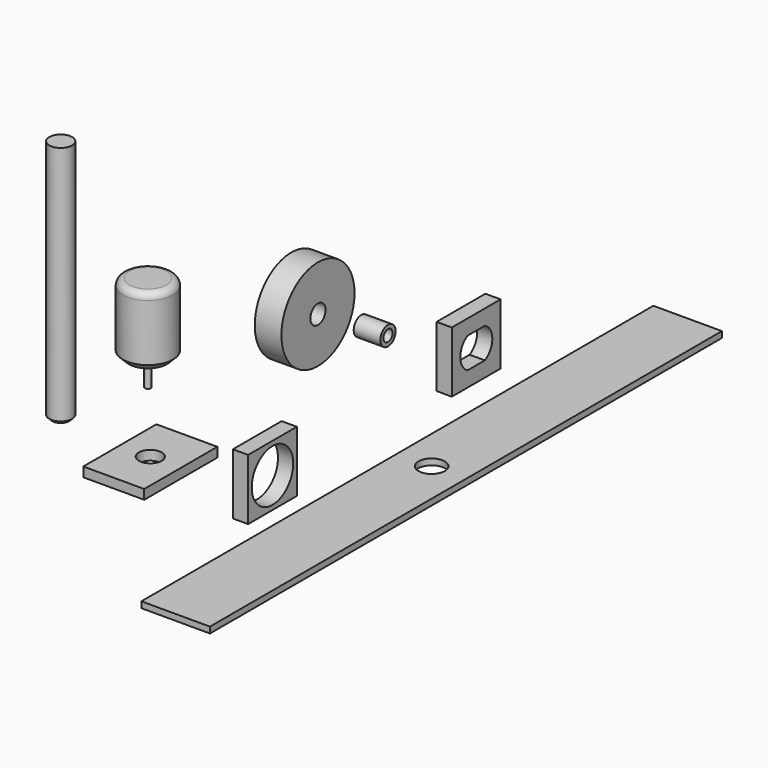
from build123d import *

# Parameters (mm, degrees)
F0_W      = 533.4
F0_H      = 5.08
F1_DEPTH  = 57.15
F2_R      = 25
F3_DEPTH  = 55
F4_SIZE   = 5.08
F5_R      = 3
F6_DEPTH  = 19.05
F7_R      = 7.9375
F7_R_2    = 4.7625
F8_DEPTH  = 22.225
F9_R      = 38.1
F9_R_2    = 7.9375
F10_DEPTH = 22.225
F11_R     = 10.9718927616
F12_DEPTH = 25.4
F14_R     = 21
F15_DEPTH = 58
F16_SIZE  = 5.08
F17_R     = 5.588
F18_R     = 2.5
F19_DEPTH = 22
F20_W     = 50.8
F20_H     = 50.8
F20_R     = 21.59
F21_DEPTH = 12.7
F22_W     = 50.8
F22_H     = 50.8
F23_DEPTH = 12.7
F24_W     = 50.8
F24_H     = 76.2
F24_R     = 9.525
F25_DEPTH = 7.9375
F26_R     = 9.525
F27_DEPTH = 203.2
F28_SIZE  = 2.54


# Not quite as in the source:
# - a length typed as a fraction of an inch, garbled in the dataset ("3 / 203.2 mm" for 3/8 in), is restored


with BuildPart() as f1:
    # F0 (on Right) → F1 (new body)
    with BuildSketch(Plane.YZ):
        with Locations((65.3649564266, -16.4303069627)):
            Rectangle(F0_W, F0_H)
    extrude(amount=F1_DEPTH)

    # F11 (on face) → F12 (cut)
    with BuildSketch(Plane.XY.offset(-13.8903069627)):
        with Locations((28.575, 65.3649564266)):
            Circle(F11_R)
    extrude(amount=-F12_DEPTH, mode=Mode.SUBTRACT)


with BuildPart() as f3:
    # F2 (on Top) → F3 (new body)
    with BuildSketch(Plane.XY):
        with Locations((-105.339050293, -53.4889884293)):
            Circle(F2_R)
    extrude(amount=F3_DEPTH)

    # F4
    f4_edges = [f3.edges().sort_by_distance(p)[0] for p in [
        (-130.33905, -53.488988, 55),
    ]]
    chamfer(f4_edges, length=F4_SIZE)

    # F5 (on face) → F6 (join)
    with BuildSketch(Plane(origin=(0, 0, 0), x_dir=(1, 0, 0), z_dir=(0, 0, -1))):
        with Locations((-105.339050293, 53.4889884293)):
            Circle(F5_R)
    extrude(amount=F6_DEPTH)


with BuildPart() as f8:
    # F7 (on Right) → F8 (new body)
    with BuildSketch(Plane.YZ):
        with Locations((27.8154350817, 95.117174089)):
            Circle(F7_R)
        with Locations((27.8154350817, 95.117174089)):
            Circle(F7_R_2, mode=Mode.SUBTRACT)
    extrude(amount=F8_DEPTH)


with BuildPart() as f10:
    # F9 (on Right) → F10 (new body)
    with BuildSketch(Plane.YZ):
        with Locations((-45.1477132738, 140.5126005411)):
            Circle(F9_R)
        with Locations((-45.1477132738, 140.5126005411)):
            Circle(F9_R_2, mode=Mode.SUBTRACT)
    extrude(amount=F10_DEPTH)


with BuildPart() as f15:
    # F14 (on Top) → F15 (new body)
    with BuildSketch(Plane.XY):
        with Locations((-194.9862390757, 49.1990633309)):
            Circle(F14_R)
    extrude(amount=F15_DEPTH)

    # F16
    f16_edges = [f15.edges().sort_by_distance(p)[0] for p in [
        (-215.986239, 49.199063, 0),
    ]]
    chamfer(f16_edges, length=F16_SIZE)

    # F17
    f17_edges = [f15.edges().sort_by_distance(p)[0] for p in [
        (-215.986239, 49.199063, 58),
    ]]
    fillet(f17_edges, radius=F17_R)

    # F18 (on face) → F19 (join)
    with BuildSketch(Plane(origin=(0, 0, 0), x_dir=(1, 0, 0), z_dir=(0, 0, -1))):
        with Locations((-194.9862390757, -49.1990633309)):
            Circle(F18_R)
    extrude(amount=F19_DEPTH)


with BuildPart() as f21:
    # F20 (on Right) → F21 (new body)
    with BuildSketch(Plane.YZ):
        with Locations((-80.6285493731, 33.508805865)):
            Rectangle(F20_W, F20_H)
        with Locations((-80.6285493731, 33.508805865)):
            Circle(F20_R, mode=Mode.SUBTRACT)
    extrude(amount=F21_DEPTH)


with BuildPart() as f23:
    # F22 (on Right) → F23 (new body)
    with BuildSketch(Plane.YZ):
        with Locations((131.6323596907, 40.7181175649)):
            Rectangle(F22_W, F22_H)
        with BuildLine():
            Line((122.6420296907, 53.4181175649), (140.6226896907, 53.4181175649))
            ThreePointArc((140.6226896907, 53.4181175649), (148.4102478202, 40.7181175649), (140.6226896907, 28.0181175649))
            Line((140.6226896907, 28.0181175649), (122.6420296907, 28.0181175649))
            ThreePointArc((122.6420296907, 28.0181175649), (115.0493723243, 40.7181175649), (122.6420296907, 53.4181175649))
        make_face(mode=Mode.SUBTRACT)
    extrude(amount=F23_DEPTH)


with BuildPart() as f25:
    # F24 (on Top) → F25 (new body)
    with BuildSketch(Plane.XY):
        with Locations((-96.6411658287, -71.230996871)):
            Rectangle(F24_W, F24_H)
        with Locations((-96.6411658287, -71.230996871)):
            Circle(F24_R, mode=Mode.SUBTRACT)
    extrude(amount=F25_DEPTH)


with BuildPart() as f27:
    # F26 (on Top) → F27 (new body)
    with BuildSketch(Plane.XY):
        with Locations((-185.5818331242, -53.4064434469)):
            Circle(F26_R)
    extrude(amount=F27_DEPTH)

    # F28
    f28_edges = [f27.edges().sort_by_distance(p)[0] for p in [
        (-195.106833, -53.406443, 0),
    ]]
    chamfer(f28_edges, length=F28_SIZE)


solid = Compound([f1.part, f8.part, f10.part, f15.part, f21.part, f23.part, f25.part, f27.part])
